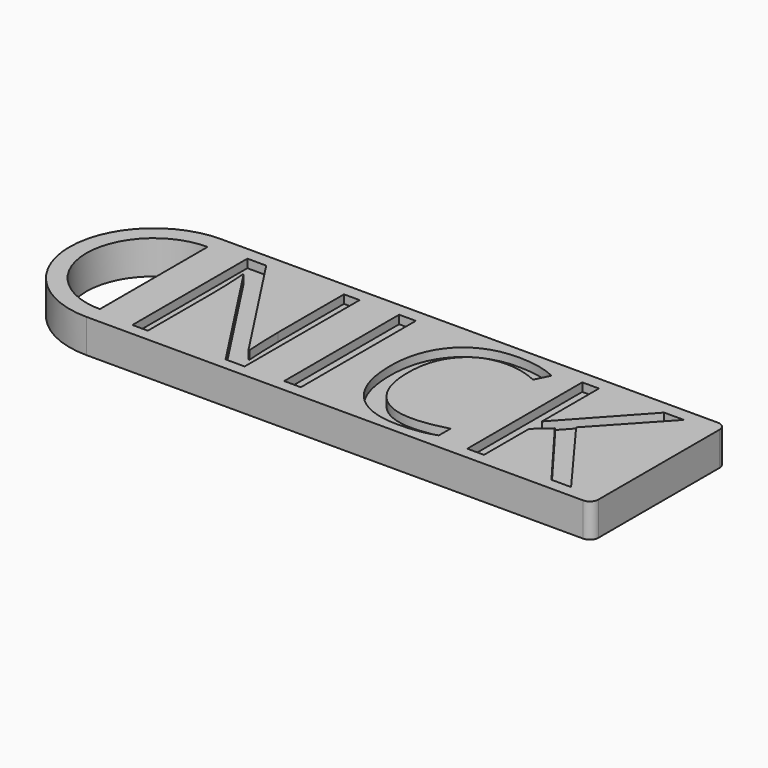
from build123d import *

# Parameters (mm, degrees)
F4_DEPTH     = 2
F1_R         = 0.5
F2_TEXT_SIZE = 11.9546364243
F3_DEPTH     = 0.5


# Not quite as in the source:
# - Text() gives the source's letters only with a copy of the font that has no kerning and outlines rounded to 1/6400 em; it was checked with that copy


with BuildPart() as f4:
    # F0 (on Top) → F4 (new body)
    with BuildSketch(Plane.XY):
        Polygon((24.7291392038, 3.2207785361), (-5.2708607962, 3.2207785361), (-5.2708607962, 2.2207785361), (-5.2708607962, -5.7792214639), (-5.2708607962, -6.7792214639), (24.7291392038, -6.7792214639), align=None)
        with BuildLine():
            Line((-5.2708607962, 2.2207785361), (-5.2708607962, 3.2207785361))
            ThreePointArc((-5.2708607962, 3.2207785361), (-10.2708607962, -1.7792214639), (-5.2708607962, -6.7792214639))
            Line((-5.2708607962, -6.7792214639), (-5.2708607962, -5.7792214639))
            ThreePointArc((-5.2708607962, -5.7792214639), (-9.2708607962, -1.7792214639), (-5.2708607962, 2.2207785361))
        make_face()
    extrude(amount=F4_DEPTH)

    # F1
    f1_edges = [f4.edges().sort_by_distance(p)[0] for p in [
        (24.729139, -6.779221, 1),
        (24.729139, 3.220779, 1),
    ]]
    fillet(f1_edges, radius=F1_R)

    # F2 (on face) → F3 (cut)
    with BuildSketch(Plane.XY.offset(2)):
        with Locations((-4.2708607962, -6.0828905767)):
            Text('NICK', F2_TEXT_SIZE, font='Open Sans', text_align=(TextAlign.LEFT, TextAlign.BOTTOM))
    extrude(amount=-F3_DEPTH, mode=Mode.SUBTRACT)


solid = f4.part
